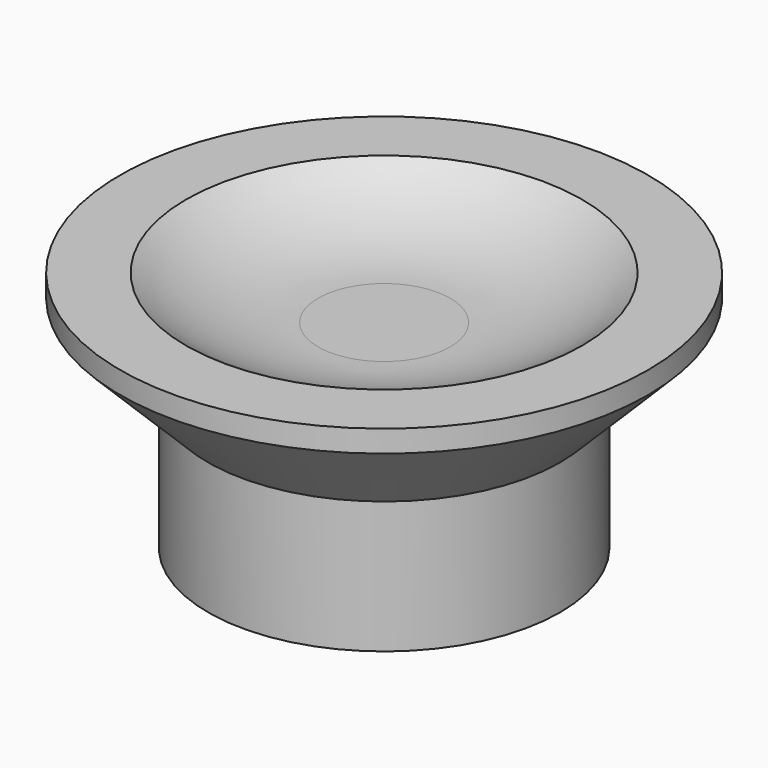
from build123d import *

# Parameters (mm, degrees)
F0_R     = 4
F1_DEPTH = 3
F2_R     = 6
F3_DEPTH = 2.5
F4_SIZE  = 1.99999
F5_R     = 4.5
F6_DEPTH = 1


# Not quite as in the source:
# - a fillet or chamfer that OpenCascade refuses, or shapes differently, is made with other operations: its cross-section is extruded or revolved along the edge and cut away or added
# - a fillet or chamfer is up to 0.001 mm smaller than in the source, because OpenCascade refuses the exact size


with BuildPart() as f1:
    # F0 (on Top) → F1 (new body)
    with BuildSketch(Plane.XY):
        Circle(F0_R)
    extrude(amount=F1_DEPTH)

    # F2 (on face) → F3 (join)
    with BuildSketch(Plane.XY.offset(3)):
        Circle(F2_R)
    extrude(amount=F3_DEPTH)

    # F4 (size 2 in the source; OpenCascade refuses exactly that, so slightly less here)
    f4_edges = [f1.edges().sort_by_distance(p)[0] for p in [
        (-6, 0, 3),
    ]]
    chamfer(f4_edges, length=F4_SIZE)

    # F5 (on face) → F6 (cut)
    with BuildSketch(Plane.XY.offset(5.5)):
        Circle(F5_R)
    extrude(amount=-F6_DEPTH, mode=Mode.SUBTRACT)

    # F7: fillet of radius 5 on 1 edges, made by hand

    # F7_s1 → F7_t2 (revolve)
    with BuildSketch(Plane.XZ):
        with BuildLine():
            ThreePointArc((4.5, 5.5), (3.0811388301, 4.7565835097), (1.5, 4.5))
            Line((1.5, 4.5), (4.5, 4.5))
            Line((4.5, 4.5), (4.5, 5.5))
        make_face()
    revolve(axis=Axis((0, 0, 4.5), (0, 0, 1)))


solid = f1.part
